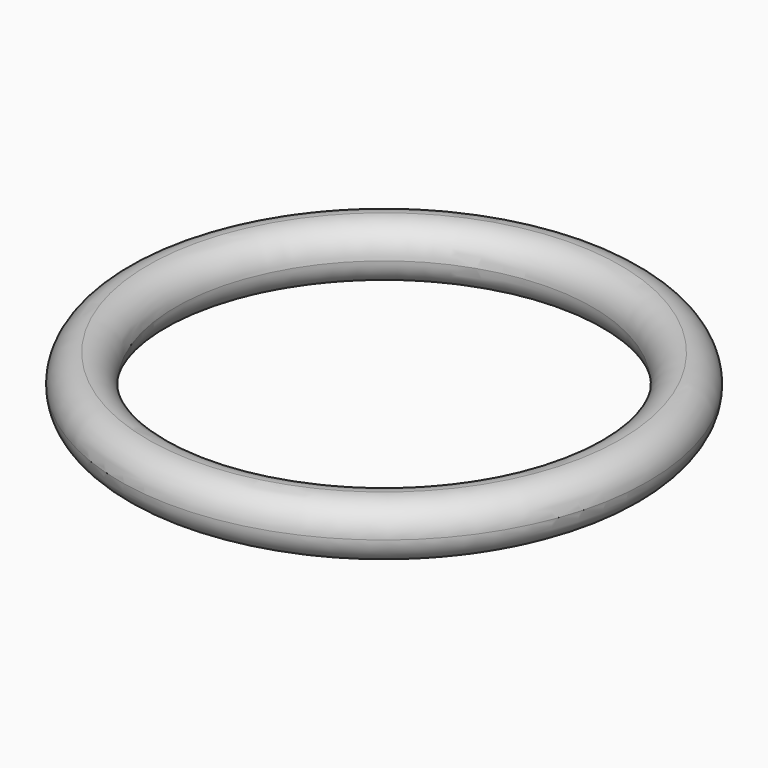
from build123d import *

# Parameters (mm, degrees)
F0_R     = 9.5
F0_R_2   = 7.5
F1_DEPTH = 2
F2_R     = 0.99999


# Not quite as in the source:
# - a fillet or chamfer is up to 0.001 mm smaller than in the source, because OpenCascade refuses the exact size


with BuildPart() as f1:
    # F0 (on Top) → F1 (new body)
    with BuildSketch(Plane.XY):
        Circle(F0_R)
        Circle(F0_R_2, mode=Mode.SUBTRACT)
    extrude(amount=F1_DEPTH)

    # F2 (radius 1 in the source; OpenCascade refuses exactly that, so slightly less here)
    f2_edges = [f1.edges().sort_by_distance(p)[0] for p in [
        (-9.5, 0, 2),
        (-9.5, 0, 0),
        (-7.5, 0, 2),
        (-7.5, 0, 0),
    ]]
    fillet(f2_edges, radius=F2_R)


solid = f1.part
